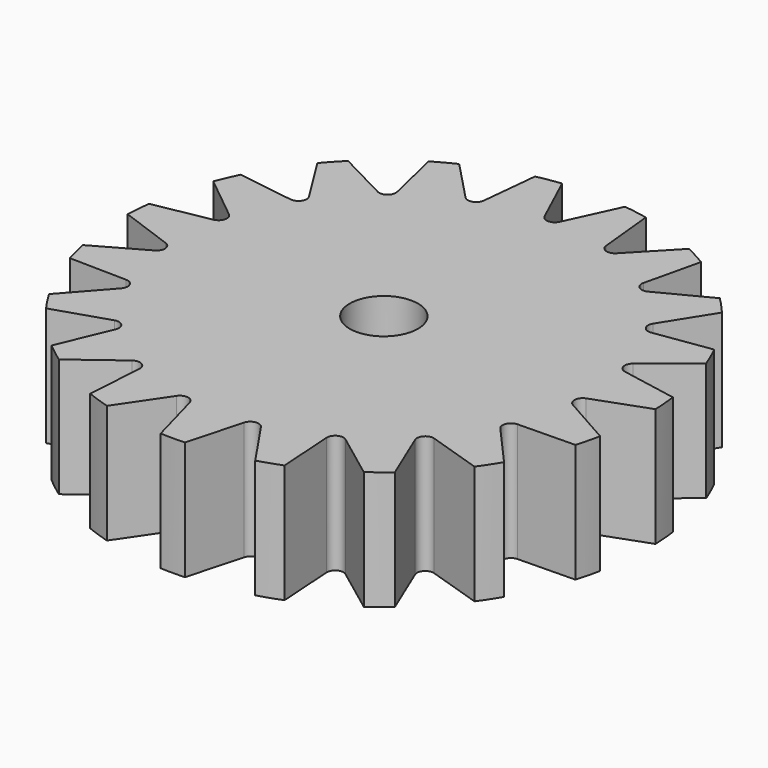
from build123d import *

# Parameters (mm, degrees)
F0_R            = 14.1331511128
F0_R_2          = 1.8288
F1_DEPTH        = 6.35
F2_W            = 9.1077039159
F2_H            = 9.1077039159
F3_DEPTH        = 3.175
F4_R            = 6.4401192
F5_DEPTH        = 1.5875
F7_DEPTH        = 6.35
F7_COPIES_COUNT = 19


# Not quite as in the source:
# - a pattern or mirror of a feature is missing from the dataset's text; its kind, count and spacing are read off the source's solid


with BuildPart() as f1:
    # F0 (on Top) → F1 (new body)
    with BuildSketch(Plane.XY):
        Circle(F0_R)
        Circle(F0_R_2, mode=Mode.SUBTRACT)
    extrude(amount=F1_DEPTH)

    # F2 (on face) → F3 (cut)
    with BuildSketch(Plane(origin=(0, 0, 0), x_dir=(1, 0, 0), z_dir=(0, 0, -1))):
        Rectangle(F2_W, F2_H)
    extrude(amount=-F3_DEPTH, mode=Mode.SUBTRACT)

    # F4 (on face) → F5 (cut)
    with BuildSketch(Plane(origin=(0, 0, 0), x_dir=(1, 0, 0), z_dir=(0, 0, -1))):
        Circle(F4_R)
    extrude(amount=-F5_DEPTH, mode=Mode.SUBTRACT)

    # F6 (on face) → F7 (cut, through all)
    with BuildSketch(Plane.XY.offset(6.35)):
        with BuildLine():
            Line((0.4054121916, 11.2582715851), (1.6826301613, 14.0326304063))
            ThreePointArc((1.6826301613, 14.0326304063), (0, 14.1331511128), (-1.6826301613, 14.0326304063))
            Line((-1.6826301613, 14.0326304063), (-0.4054121916, 11.2582715851))
            ThreePointArc((-0.4054121916, 11.2582715851), (0, 10.9985991732), (0.4054121916, 11.2582715851))
        make_face()
    f7 = extrude(amount=-F7_DEPTH, mode=Mode.SUBTRACT)

    # F7_copies: F7 ×19 about axis
    f7_copies_axis = Axis((0, 0, 0), (0, 0, 1))
    for i in range(1, F7_COPIES_COUNT):
        add(f7.rotate(f7_copies_axis, i * 360 / F7_COPIES_COUNT), mode=Mode.SUBTRACT)


solid = f1.part
